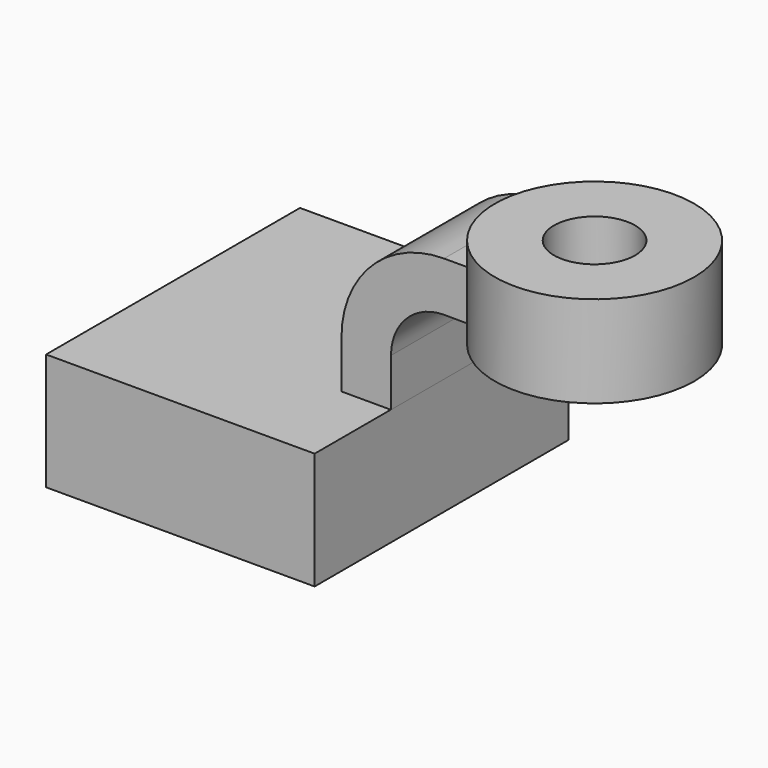
from build123d import *

# Parameters (mm, degrees)
F1_DEPTH = 63.5
F2_DEPTH = 25.4
F0_W     = 39.8683473468
F0_H     = 36.688753669
F4_R     = 16.2187232802
F5_DEPTH = 36.688753669


with BuildPart() as f1:
    # F0 (on Front) → F1 (new body, symmetric)
    with BuildSketch(Plane.XZ):
        Polygon((-53.7355877459, -23.4009865671), (53.7355877459, -23.4009865671), (53.7355877459, 23.4009865671), (34.0091888793, 23.4009865671), (-53.7355877459, 23.4009865671), align=None)
    extrude(amount=F1_DEPTH, both=True)


with BuildPart() as f2:
    # F0 (on Front) → F2 (new body, symmetric)
    with BuildSketch(Plane.XZ):
        with BuildLine():
            Line((34.0091888793, 23.4009865671), (53.7355877459, 23.4009865671))
            Line((53.7355877459, 23.4009865671), (53.821187932, 23.4009865671))
            Line((53.821187932, 23.4009865671), (53.821187932, 42.5507634298))
            ThreePointArc((53.821187932, 42.5507634298), (60.0390651231, 57.5620468738), (75.0503485671, 63.7799240649))
            Line((75.0503485671, 63.7799240649), (75.096371118, 63.7799240649))
            Line((75.096371118, 63.7799240649), (75.096371118, 83.5919231176))
            Line((75.096371118, 83.5919231176), (75.0503485671, 83.5919231176))
            ThreePointArc((75.0503485671, 83.5919231176), (46.0298662441, 71.5712457528), (34.0091888793, 42.5507634298))
            Line((34.0091888793, 42.5507634298), (34.0091888793, 23.4009865671))
        make_face()
        Polygon((93.9475916658, 83.5919231176), (75.096371118, 83.5919231176), (75.096371118, 63.7799240649), (93.9475916658, 63.6981888188), align=None)
    extrude(amount=F2_DEPTH, both=True)


with BuildPart() as f3:
    # F0 (on Front) → F3 (revolve)
    with BuildSketch(Plane.XZ):
        with Locations((134.8988921382, 74.2934830487)):
            Rectangle(F0_W, F0_H)
    revolve(axis=Axis((114.9647184648, 0, 74.2934830487), (0, 0, 1)))

    # F4 (on face) → F5 (cut, through all)
    with BuildSketch(Plane.XY.offset(92.6378598832)):
        with Locations((114.9647184648, 0)):
            Circle(F4_R)
    extrude(amount=-F5_DEPTH, mode=Mode.SUBTRACT)


solid = Compound([f1.part, f2.part, f3.part])
